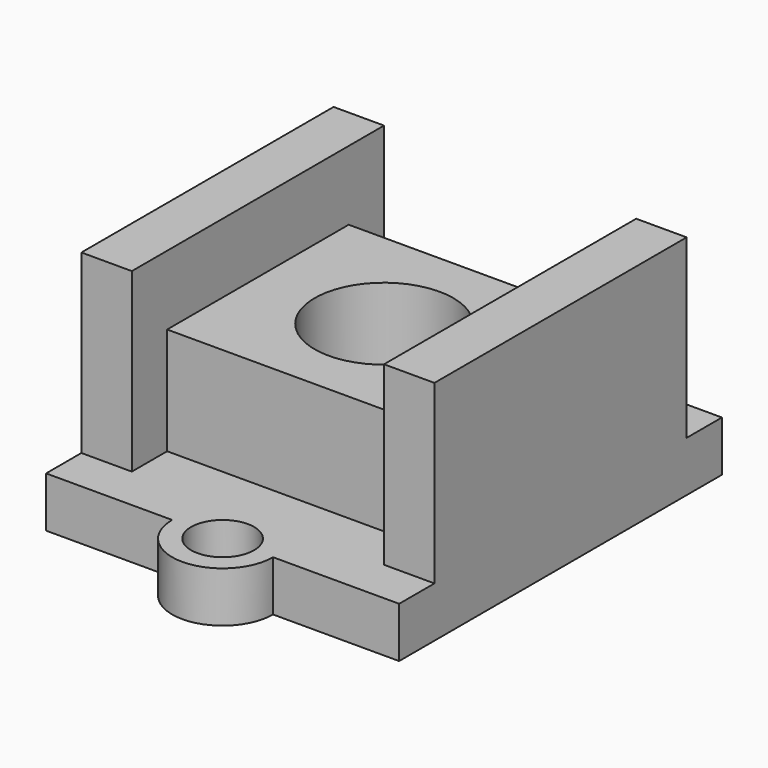
from build123d import *

# Parameters (mm, degrees)
F0_W      = 56
F0_H      = 64
F1_DEPTH  = 8
F2_W      = 8
F2_H      = 50
F3_DEPTH  = 28
F4_R      = 8
F5_DEPTH  = 8
F6_R      = 5
F7_DEPTH  = 8.001
F8_W      = 40
F8_H      = 36
F9_DEPTH  = 17
F10_R     = 11
F11_DEPTH = 25.001


# Not quite as in the source:
# - a pattern or mirror of a feature is missing from the dataset's text; its kind, count and spacing are read off the source's solid


with BuildPart() as f1:
    # F0 (on Top) → F1 (new body)
    with BuildSketch(Plane.XY):
        Rectangle(F0_W, F0_H)
    extrude(amount=-F1_DEPTH)

    # F2 (on face) → F3 (join)
    with BuildSketch(Plane.XY):
        with Locations((-24, 0)):
            Rectangle(F2_W, F2_H)
    f3 = extrude(amount=F3_DEPTH)

    # F3_copies: F3 across plane
    add(f3.mirror(Plane(origin=(0, 0, 0), x_dir=(0, 0, 1), z_dir=(1, 0, 0))))

    # F4 (on face) → F5 (join, through all)
    with BuildSketch(Plane.XY):
        with Locations((0, -32)):
            Circle(F4_R)
    f5 = extrude(amount=-F5_DEPTH)

    # F5_copies: F5 across plane
    add(f5.mirror(Plane.ZX))

    # F6 (on face) → F7 (cut, through all)
    with BuildSketch(Plane.XY):
        with Locations((0, -32)):
            Circle(F6_R)
    f7 = extrude(amount=-F7_DEPTH, mode=Mode.SUBTRACT)

    # F7_copies: F7 across plane
    add(f7.mirror(Plane.ZX), mode=Mode.SUBTRACT)

    # F8 (on face) → F9 (join)
    with BuildSketch(Plane.XY):
        Rectangle(F8_W, F8_H)
    extrude(amount=F9_DEPTH)

    # F10 (on face) → F11 (cut, through all)
    with BuildSketch(Plane.XY.offset(17)):
        Circle(F10_R)
    extrude(amount=-F11_DEPTH, mode=Mode.SUBTRACT)


solid = f1.part
